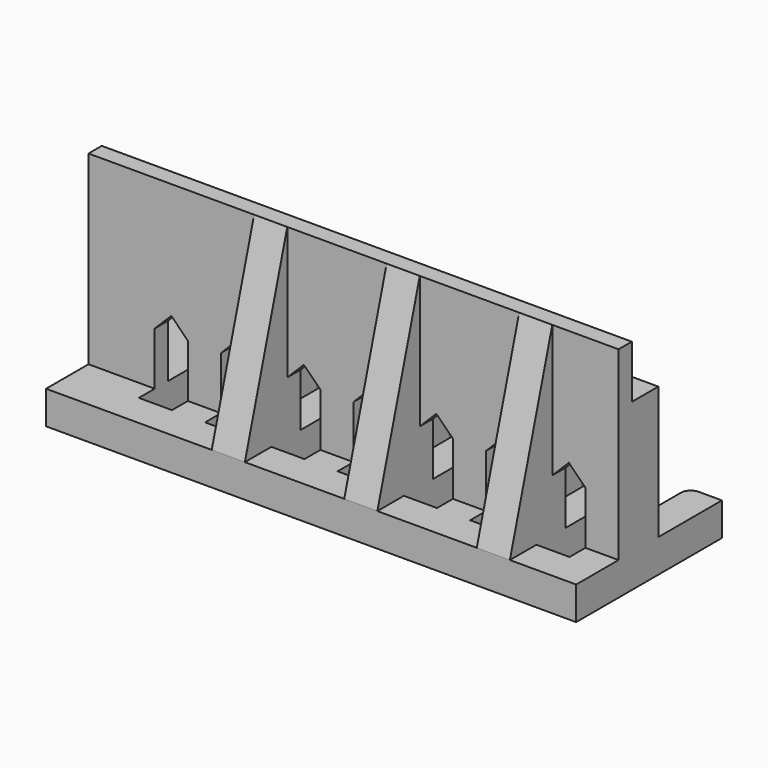
from build123d import *

# Parameters (mm, degrees)
F0_W      = 12.7
F0_H      = 57.15
F1_DEPTH  = 12.7
F2_W      = 25.4
F2_H      = 6.35
F2_W_2    = 12.7
F3_DEPTH  = 20.32
F4_W      = 25.4
F4_H      = 6.35
F4_W_2    = 12.7
F5_DEPTH  = 50.8
F6_W      = 12.7
F6_H      = 50.8
F7_DEPTH  = 12.7
F9_DEPTH  = 12.7
F11_DEPTH = 12.7
F13_DEPTH = 12.7
F14_W     = 12.7
F14_H     = 50.8
F15_DEPTH = 12.7
F16_R     = 3.81
F18_DEPTH = 6.35
F19_R     = 3.81


# Not quite as in the source:
# - a feature names something its author has since deleted; it is built from what else it names


with BuildPart() as f1:
    # F0 (on Top) → F1 (new body)
    with BuildSketch(Plane.XY):
        Polygon((101.6, -34.925), (101.6, 34.925), (88.9, 34.925), (88.9, -22.225), (76.2, -22.225), (76.2, 34.925), (63.5, 34.925), (63.5, -22.225), (50.8, -22.225), (50.8, 34.925), (38.1, 34.925), (38.1, -22.225), (25.4, -22.225), (25.4, 34.925), (12.7, 34.925), (12.7, -22.225), (0, -22.225), (0, 34.925), (-12.7, 34.925), (-12.7, -22.225), (-25.4, -22.225), (-25.4, 34.925), (-38.1, 34.925), (-38.1, -22.225), (-50.8, -22.225), (-50.8, 34.925), (-63.5, 34.925), (-63.5, -22.225), (-76.2, -22.225), (-76.2, 34.925), (-88.9, 34.925), (-88.9, -22.225), (-101.6, -22.225), (-101.6, -34.925), align=None)
        with Locations((-95.25, 6.35)):
            Rectangle(F0_W, F0_H)
    extrude(amount=F1_DEPTH)

    # F2 (on face) → F3 (join)
    with BuildSketch(Plane.XY.offset(12.7)):
        with Locations((-88.9, -11.43)):
            Rectangle(F2_W, F2_H)
        with Locations((-31.75, -11.43)):
            Rectangle(F2_W_2, F2_H)
        with Locations((-6.35, -11.43)):
            Rectangle(F2_W_2, F2_H)
        with Locations((19.05, -11.43)):
            Rectangle(F2_W_2, F2_H)
        with Locations((44.45, -11.43)):
            Rectangle(F2_W_2, F2_H)
        with Locations((69.85, -11.43)):
            Rectangle(F2_W_2, F2_H)
        with Locations((95.25, -11.43)):
            Rectangle(F2_W_2, F2_H)
        with Locations((-57.15, -11.43)):
            Rectangle(F2_W_2, F2_H)
    extrude(amount=F3_DEPTH)

    # F4 (on face) → F5 (join)
    with BuildSketch(Plane.XY.offset(33.02)):
        with Locations((-88.9, -11.43)):
            Rectangle(F4_W, F4_H)
        with Locations((-69.85, -11.43)):
            Rectangle(F4_W_2, F4_H)
        with Locations((-57.15, -11.43)):
            Rectangle(F4_W_2, F4_H)
        with Locations((-44.45, -11.43)):
            Rectangle(F4_W_2, F4_H)
        with Locations((-31.75, -11.43)):
            Rectangle(F4_W_2, F4_H)
        with Locations((-19.05, -11.43)):
            Rectangle(F4_W_2, F4_H)
        with Locations((-6.35, -11.43)):
            Rectangle(F4_W_2, F4_H)
        with Locations((6.35, -11.43)):
            Rectangle(F4_W_2, F4_H)
        with Locations((19.05, -11.43)):
            Rectangle(F4_W_2, F4_H)
        with Locations((31.75, -11.43)):
            Rectangle(F4_W_2, F4_H)
        with Locations((44.45, -11.43)):
            Rectangle(F4_W_2, F4_H)
        with Locations((57.15, -11.43)):
            Rectangle(F4_W_2, F4_H)
        with Locations((69.85, -11.43)):
            Rectangle(F4_W_2, F4_H)
        with Locations((82.55, -11.43)):
            Rectangle(F4_W_2, F4_H)
        with Locations((95.25, -11.43)):
            Rectangle(F4_W_2, F4_H)
    extrude(amount=F5_DEPTH)

    # F6 (on face) → F7 (join)
    with BuildSketch(Plane(origin=(-101.6, 0, 0), x_dir=(0, -1, 0), z_dir=(-1, 0, 0))):
        Polygon((8.255, 63.5), (8.255, 12.7), (-4.445, 12.7), (-34.925, 12.7), (-34.925, 0), (34.925, 0), (34.925, 12.7), (14.605, 12.7), (14.605, 83.82), (8.255, 83.82), align=None)
        with Locations((1.905, 38.1)):
            Rectangle(F6_W, F6_H)
    extrude(amount=-F7_DEPTH)

    # F8 (on face) → F9 (join, through all)
    with BuildSketch(Plane.YZ.offset(-25.4)):
        Polygon((-14.605, 33.02), (-14.605, 83.82), (-34.925, 12.7), (-22.225, 12.7), (-14.605, 12.7), align=None)
    extrude(amount=-F9_DEPTH)

    # F10 (on face) → F11 (join, through all)
    with BuildSketch(Plane.YZ.offset(25.4)):
        Polygon((-14.605, 33.02), (-14.605, 83.82), (-34.925, 12.7), (-22.225, 12.7), (-14.605, 12.7), align=None)
    extrude(amount=-F11_DEPTH)

    # F12 (on face) → F13 (join, through all)
    with BuildSketch(Plane.YZ.offset(76.2)):
        Polygon((-14.605, 33.02), (-14.605, 83.82), (-34.925, 12.7), (-22.225, 12.7), (-14.605, 12.7), align=None)
    extrude(amount=-F13_DEPTH)

    # F14 (on face) → F15 (join, through all)
    with BuildSketch(Plane.YZ.offset(101.6)):
        with Locations((-1.905, 38.1)):
            Rectangle(F14_W, F14_H)
    extrude(amount=-F15_DEPTH)

    # F16
    f16_edges = [f1.edges().sort_by_distance(p)[0] for p in [
        (88.9, 34.925, 6.35),
        (63.5, 34.925, 6.35),
        (38.1, 34.925, 6.35),
        (12.7, 34.925, 6.35),
        (-12.7, 34.925, 6.35),
        (-38.1, 34.925, 6.35),
        (76.2, 34.925, 6.35),
        (50.8, 34.925, 6.35),
        (25.4, 34.925, 6.35),
        (0, 34.925, 6.35),
        (-25.4, 34.925, 6.35),
        (-50.8, 34.925, 6.35),
        (-76.2, 34.925, 6.35),
        (-63.5, 34.925, 6.35),
    ]]
    fillet(f16_edges, radius=F16_R)

    # F17 (on face) → F18 (cut, through all)
    with BuildSketch(Plane.XZ.offset(14.605)):
        Polygon((-44.45, 39.37), (-50.8, 33.02), (-38.1, 33.02), align=None)
        Polygon((-25.4, 33.02), (-12.7, 33.02), (-19.05, 39.37), align=None)
        Polygon((6.35, 39.37), (0, 33.02), (12.7, 33.02), align=None)
        Polygon((31.75, 39.37), (25.4, 33.02), (38.1, 33.02), align=None)
        Polygon((57.15, 39.37), (50.8, 33.02), (63.5, 33.02), align=None)
        Polygon((76.2, 33.02), (88.9, 33.02), (82.55, 39.37), align=None)
        Polygon((-76.2, 33.02), (-63.5, 33.02), (-69.85, 39.37), align=None)
    extrude(amount=-F18_DEPTH, mode=Mode.SUBTRACT)

    # F19
    f19_edges = [f1.edges().sort_by_distance(p)[0] for p in [
        (-88.9, 4.445, 38.1),
        (88.9, 4.445, 38.1),
    ]]
    fillet(f19_edges, radius=F19_R)


solid = f1.part
